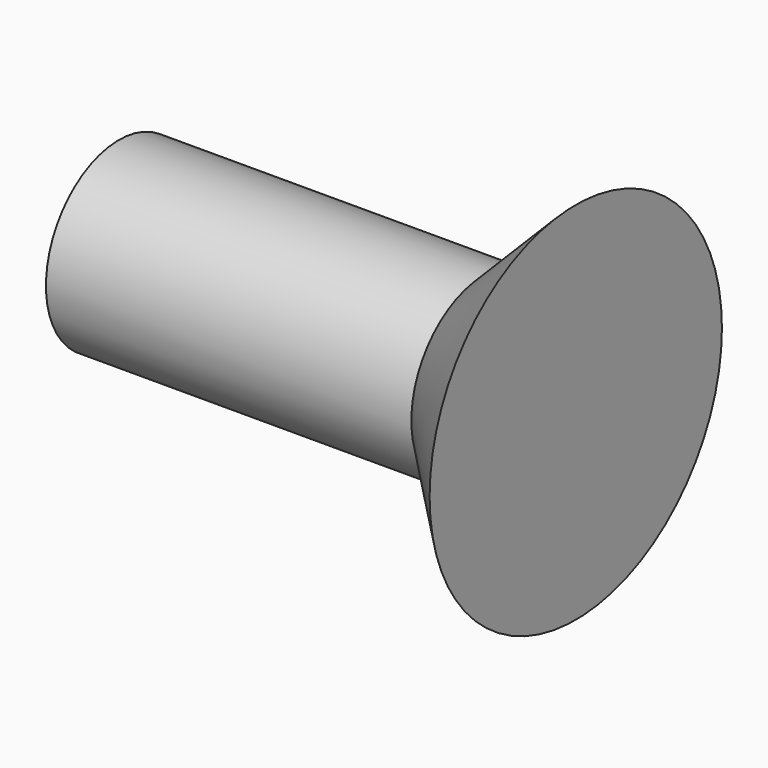
from build123d import *

# Parameters (mm, degrees)
F0_R     = 3
F1_DEPTH = 15
F2_R     = 6
F2_R_2   = 3
F3_DEPTH = 3
F4_SIZE  = 2.99999


# Not quite as in the source:
# - a fillet or chamfer is up to 0.001 mm smaller than in the source, because OpenCascade refuses the exact size


with BuildPart() as f1:
    # F0 (on Right) → F1 (new body)
    with BuildSketch(Plane.YZ):
        Circle(F0_R)
    extrude(amount=F1_DEPTH)

    # F2 (on face) → F3 (join)
    with BuildSketch(Plane.YZ.offset(15)):
        Circle(F2_R)
        Circle(F2_R_2, mode=Mode.SUBTRACT)
    extrude(amount=-F3_DEPTH)

    # F4 (size 3 in the source; OpenCascade refuses exactly that, so slightly less here)
    f4_edges = [f1.edges().sort_by_distance(p)[0] for p in [
        (12, -6, 0),
    ]]
    chamfer(f4_edges, length=F4_SIZE)


solid = f1.part
